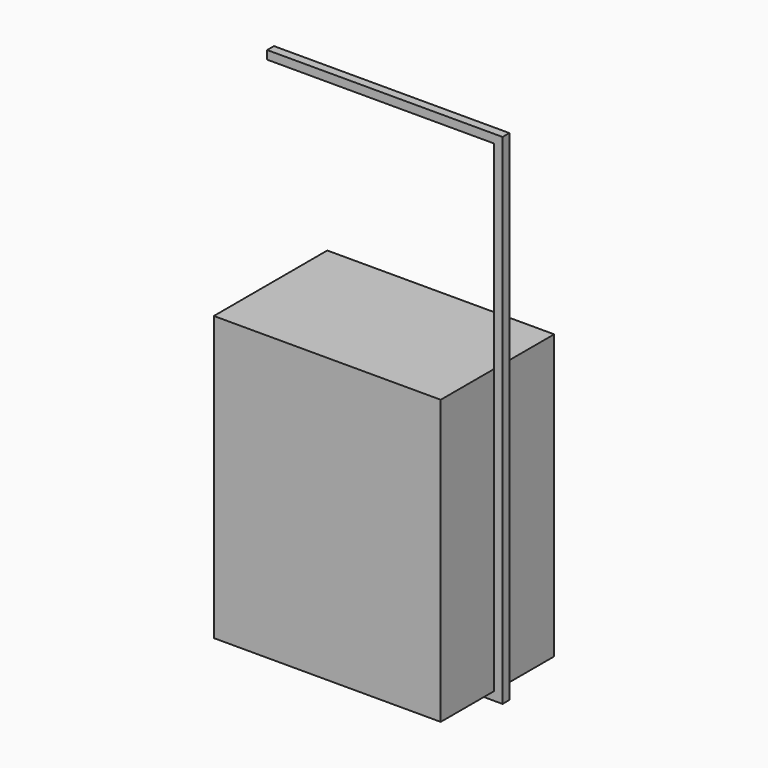
from build123d import *

# Parameters (mm, degrees)
F0_W     = 800
F0_H     = 500
F1_DEPTH = 1000
F3_DEPTH = 15
F4_W     = 600
F4_H     = 300
F4_W_2   = 540
F4_H_2   = 240
F5_DEPTH = 30


with BuildPart() as f1:
    # F0 (on Top) → F1 (new body)
    with BuildSketch(Plane.XY):
        Rectangle(F0_W, F0_H)
    extrude(amount=F1_DEPTH)


with BuildPart() as f3:
    # F2 (on Front) → F3 (new body, symmetric)
    with BuildSketch(Plane.XZ):
        Polygon((400, 1700), (400, 0), (-400, 0), (-400, -30), (430, -30), (430, 1730), (-400, 1730), (-400, 1700), align=None)
    extrude(amount=F3_DEPTH, both=True)

    # F4 (on face) → F5 (join)
    with BuildSketch(Plane(origin=(0, 0, 0), x_dir=(1, 0, 0), z_dir=(0, 0, -1))):
        Rectangle(F4_W, F4_H)
        Rectangle(F4_W_2, F4_H_2, mode=Mode.SUBTRACT)
    extrude(amount=F5_DEPTH)


solid = Compound([f1.part, f3.part])
